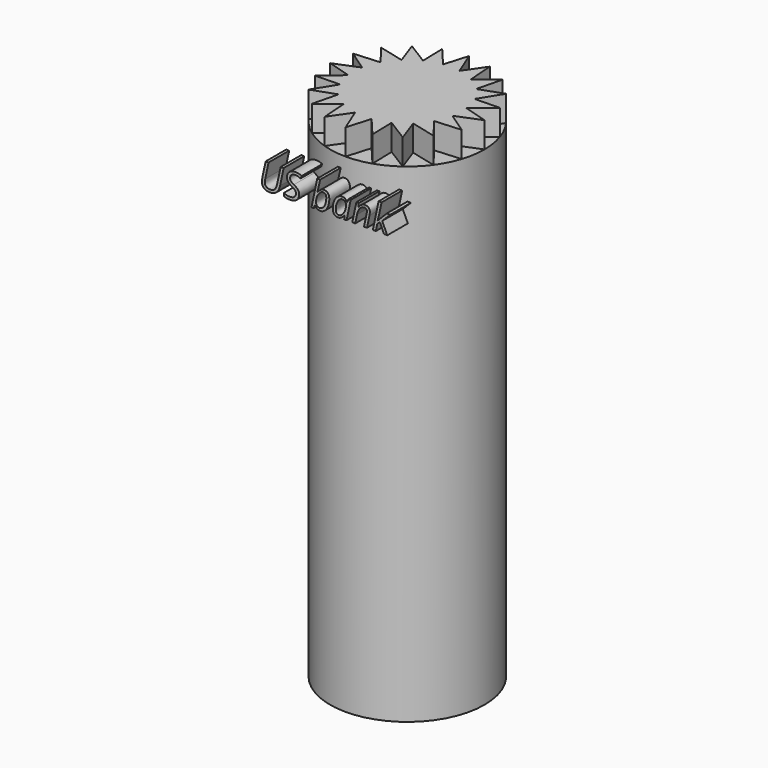
from build123d import *

# Parameters (mm, degrees)
F0_R         = 76.2
F1_DEPTH     = 508
F3_DEPTH     = 25.4
F5_TEXT_SIZE = 35.2777777778
F6_DEPTH     = 25.4


# Not quite as in the source:
# - Text() gives the source's letters only with a copy of the font that has no kerning and outlines rounded to 1/6400 em; it was checked with that copy


with BuildPart() as f1:
    # F0 (on Top) → F1 (new body)
    with BuildSketch(Plane.XY):
        Circle(F0_R)
    extrude(amount=F1_DEPTH)

    # F2 (on face) → F3 (cut)
    with BuildSketch(Plane.XY.offset(508)):
        with BuildLine():
            Line((-22.90433933, 48.0259868161), (-23.5470949714, 72.4705065417))
            ThreePointArc((-23.5470949714, 72.4705065417), (-34.5940760802, 67.8946971432), (-44.7892362247, 61.6470949714))
            Line((-44.7892362247, 61.6470949714), (-22.90433933, 48.0259868161))
        make_face()
        with BuildLine():
            Line((-6.9424750735, 52.7532578108), (0, 76.2))
            ThreePointArc((0, 76.2), (-11.9203062361, 75.2618515533), (-23.5470949714, 72.4705065417))
            Line((-23.5470949714, 72.4705065417), (-6.9424750735, 52.7532578108))
        make_face()
        with BuildLine():
            Line((9.6989670143, 52.3166723775), (23.5470949714, 72.4705065417))
            ThreePointArc((23.5470949714, 72.4705065417), (11.9203062361, 75.2618515533), (0, 76.2))
            Line((0, 76.2), (9.6989670143, 52.3166723775))
        make_face()
        with BuildLine():
            Line((25.3910066341, 46.7589665402), (44.7892362247, 61.6470949714))
            ThreePointArc((44.7892362247, 61.6470949714), (34.5940760802, 67.8946971432), (23.5470949714, 72.4705065417))
            Line((23.5470949714, 72.4705065417), (25.3910066341, 46.7589665402))
        make_face()
        with BuildLine():
            Line((38.597597615, 36.6241672691), (61.6470949714, 44.7892362247))
            ThreePointArc((61.6470949714, 44.7892362247), (53.8815367264, 53.8815367264), (44.7892362247, 61.6470949714))
            Line((44.7892362247, 61.6470949714), (38.597597615, 36.6241672691))
        make_face()
        with BuildLine():
            Line((48.0259868161, 22.90433933), (72.4705065417, 23.5470949714))
            ThreePointArc((72.4705065417, 23.5470949714), (67.8946971432, 34.5940760802), (61.6470949714, 44.7892362247))
            Line((61.6470949714, 44.7892362247), (48.0259868161, 22.90433933))
        make_face()
        with BuildLine():
            Line((72.4705065417, 23.5470949714), (52.7532578108, 6.9424750735))
            Line((52.7532578108, 6.9424750735), (76.2, 0))
            ThreePointArc((76.2, 0), (75.2618515533, 11.9203062361), (72.4705065417, 23.5470949714))
        make_face()
        with BuildLine():
            Line((76.2, 0), (52.3166723775, -9.6989670143))
            Line((52.3166723775, -9.6989670143), (72.4705065417, -23.5470949714))
            ThreePointArc((72.4705065417, -23.5470949714), (75.2618515533, -11.9203062361), (76.2, 0))
        make_face()
        with BuildLine():
            ThreePointArc((61.6470949714, -44.7892362247), (67.8946971432, -34.5940760802), (72.4705065417, -23.5470949714))
            Line((72.4705065417, -23.5470949714), (46.7589665402, -25.3910066341))
            Line((46.7589665402, -25.3910066341), (61.6470949714, -44.7892362247))
        make_face()
        with BuildLine():
            ThreePointArc((44.7892362247, -61.6470949714), (53.8815367264, -53.8815367264), (61.6470949714, -44.7892362247))
            Line((61.6470949714, -44.7892362247), (36.6241672691, -38.597597615))
            Line((36.6241672691, -38.597597615), (44.7892362247, -61.6470949714))
        make_face()
        with BuildLine():
            ThreePointArc((23.5470949714, -72.4705065417), (34.5940760802, -67.8946971432), (44.7892362247, -61.6470949714))
            Line((44.7892362247, -61.6470949714), (22.90433933, -48.0259868161))
            Line((22.90433933, -48.0259868161), (23.5470949714, -72.4705065417))
        make_face()
        with BuildLine():
            ThreePointArc((0, -76.2), (11.9203062361, -75.2618515533), (23.5470949714, -72.4705065417))
            Line((23.5470949714, -72.4705065417), (6.9424750735, -52.7532578108))
            Line((6.9424750735, -52.7532578108), (0, -76.2))
        make_face()
        with BuildLine():
            ThreePointArc((-23.5470949714, -72.4705065417), (-11.9203062361, -75.2618515533), (0, -76.2))
            Line((0, -76.2), (-9.6989670143, -52.3166723775))
            Line((-9.6989670143, -52.3166723775), (-23.5470949714, -72.4705065417))
        make_face()
        with BuildLine():
            ThreePointArc((-44.7892362247, -61.6470949714), (-34.5940760802, -67.8946971432), (-23.5470949714, -72.4705065417))
            Line((-23.5470949714, -72.4705065417), (-25.3910066341, -46.7589665402))
            Line((-25.3910066341, -46.7589665402), (-44.7892362247, -61.6470949714))
        make_face()
        with BuildLine():
            ThreePointArc((-61.6470949714, -44.7892362247), (-53.8815367264, -53.8815367264), (-44.7892362247, -61.6470949714))
            Line((-44.7892362247, -61.6470949714), (-38.597597615, -36.6241672691))
            Line((-38.597597615, -36.6241672691), (-61.6470949714, -44.7892362247))
        make_face()
        with BuildLine():
            ThreePointArc((-72.4705065417, -23.5470949714), (-67.8946971432, -34.5940760802), (-61.6470949714, -44.7892362247))
            Line((-61.6470949714, -44.7892362247), (-48.0259868161, -22.90433933))
            Line((-48.0259868161, -22.90433933), (-72.4705065417, -23.5470949714))
        make_face()
        with BuildLine():
            ThreePointArc((-76.2, 0), (-75.2618515533, -11.9203062361), (-72.4705065417, -23.5470949714))
            Line((-72.4705065417, -23.5470949714), (-52.7532578108, -6.9424750735))
            Line((-52.7532578108, -6.9424750735), (-76.2, 0))
        make_face()
        with BuildLine():
            Line((-52.3166723775, 9.6989670143), (-72.4705065417, 23.5470949714))
            ThreePointArc((-72.4705065417, 23.5470949714), (-75.2618515533, 11.9203062361), (-76.2, 0))
            Line((-76.2, 0), (-52.3166723775, 9.6989670143))
        make_face()
        with BuildLine():
            Line((-46.7589665402, 25.3910066341), (-61.6470949714, 44.7892362247))
            ThreePointArc((-61.6470949714, 44.7892362247), (-67.8946971432, 34.5940760802), (-72.4705065417, 23.5470949714))
            Line((-72.4705065417, 23.5470949714), (-46.7589665402, 25.3910066341))
        make_face()
        with BuildLine():
            Line((-36.6241672691, 38.597597615), (-44.7892362247, 61.6470949714))
            ThreePointArc((-44.7892362247, 61.6470949714), (-53.8815367264, 53.8815367264), (-61.6470949714, 44.7892362247))
            Line((-61.6470949714, 44.7892362247), (-36.6241672691, 38.597597615))
        make_face()
    extrude(amount=-F3_DEPTH, mode=Mode.SUBTRACT)

    # F5 (on offset) → F6 (join)
    with BuildSketch(Plane.XZ.offset(76.2)):
        with Locations((-65.0604276715, 444.5)):
            Text('US bank', F5_TEXT_SIZE, font='Open Sans', font_style=FontStyle.ITALIC, text_align=(TextAlign.LEFT, TextAlign.BOTTOM))
    extrude(amount=F6_DEPTH)


solid = f1.part
